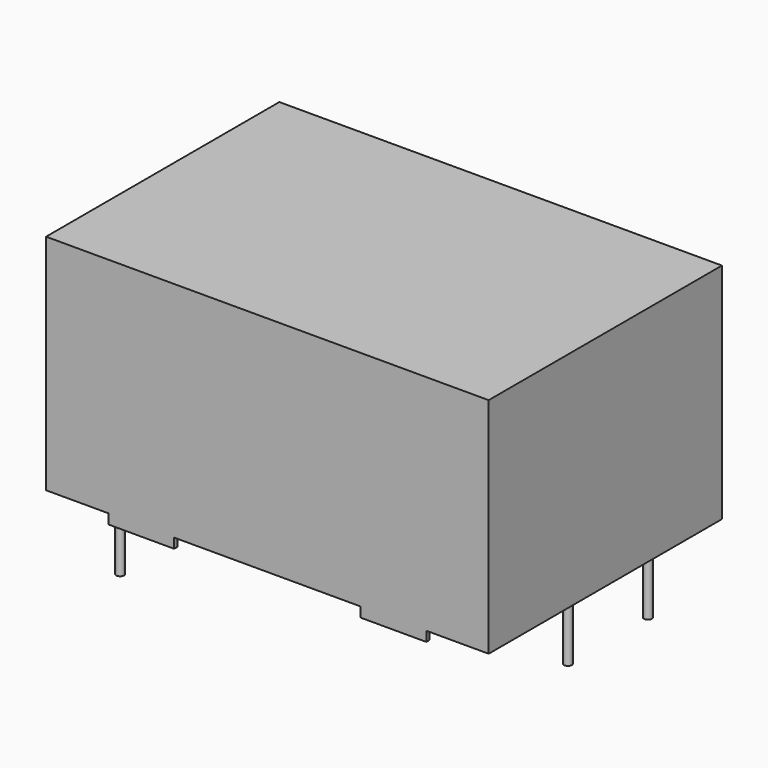
from build123d import *

# Parameters (mm, degrees)
F0_R     = 0.3
F0_W     = 5
F0_H     = 0.3
F1_DEPTH = 17
F2_DEPTH = 0.75
F3_DEPTH = 6.1


# Not quite as in the source:
# - a feature names something its author has since deleted; it is built from what else it names


with BuildPart() as f1:
    # F0 (on Top) → F1 (new body)
    with BuildSketch(Plane.XY):
        Polygon((12.1, -11.1), (16.85, -11.1), (16.85, 11.1), (12.1, 11.1), (12.1, 10.8), (7.1, 10.8), (7.1, 11.1), (-7.1, 11.1), (-7.1, 10.8), (-12.1, 10.8), (-12.1, 11.1), (-16.85, 11.1), (-16.85, -11.1), (-12.1, -11.1), (-12.1, -10.8), (-7.1, -10.8), (-7.1, -11.1), (7.1, -11.1), (7.1, -10.8), (12.1, -10.8), align=None)
        with Locations((-14, -7.62)):
            Circle(F0_R, mode=Mode.SUBTRACT)
        with Locations((-14, 7.62)):
            Circle(F0_R, mode=Mode.SUBTRACT)
        with Locations((14, 0)):
            Circle(F0_R, mode=Mode.SUBTRACT)
        with Locations((14, 7.62)):
            Circle(F0_R, mode=Mode.SUBTRACT)
        with Locations((-9.6, 10.95)):
            Rectangle(F0_W, F0_H)
        with Locations((9.6, 10.95)):
            Rectangle(F0_W, F0_H)
        with Locations((9.6, -10.95)):
            Rectangle(F0_W, F0_H)
        with Locations((-9.6, -10.95)):
            Rectangle(F0_W, F0_H)
        with Locations((-14, -7.62)):
            Circle(F0_R)
        with Locations((-14, 7.62)):
            Circle(F0_R)
        with Locations((14, 0)):
            Circle(F0_R)
        with Locations((14, 7.62)):
            Circle(F0_R)
    extrude(amount=F1_DEPTH)

    # F0 (on Top) → F2 (join)
    with BuildSketch(Plane.XY):
        with Locations((9.6, 10.95)):
            Rectangle(F0_W, F0_H)
        with Locations((-9.6, 10.95)):
            Rectangle(F0_W, F0_H)
        with Locations((-9.6, -10.95)):
            Rectangle(F0_W, F0_H)
        with Locations((9.6, -10.95)):
            Rectangle(F0_W, F0_H)
    extrude(amount=-F2_DEPTH)

    # F0 (on Top) → F3 (join)
    with BuildSketch(Plane.XY):
        with Locations((14, 0)):
            Circle(F0_R)
        with Locations((-14, 7.62)):
            Circle(F0_R)
        with Locations((-14, -7.62)):
            Circle(F0_R)
        with Locations((14, 7.62)):
            Circle(F0_R)
    extrude(amount=-F3_DEPTH)


solid = f1.part
